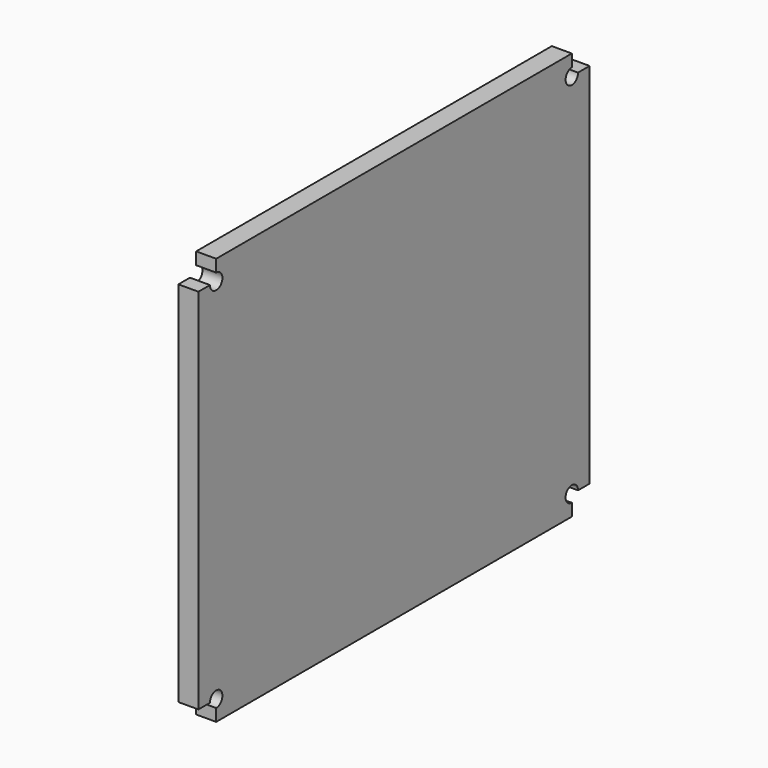
from build123d import *

# Parameters (mm, degrees)
F1_DEPTH = 9


# Not quite as in the source:
# - ends of sketch curves that miss each other by under 0.0002 mm in the source are joined


with BuildPart() as f1:
    # F0 (on Right) → F1 (new body)
    with BuildSketch(Plane.YZ):
        with BuildLine():
            Line((-71.5472308397, 116.6226820285), (-78.0472308397, 116.6226820285))
            Line((-78.0472308397, 116.6226820285), (-78.0472319707, -48.8313179715))
            Line((-78.0472319707, -48.8313179715), (-71.5472308397, -48.8313179715))
            ThreePointArc((-71.5472308397, -48.8313179715), (-65.5723571056, -46.3564442373), (-68.0472308397, -52.3313179715))
            Line((-68.0472308397, -52.3313179715), (-68.0472308397, -57.8313179715))
            Line((-68.0472308397, -57.8313179715), (31.9527691603, -57.8313179715))
            Line((31.9527691603, -57.8313179715), (131.9527668982, -57.8313179715))
            Line((131.9527668982, -57.8313179715), (131.9527668982, -52.3313179715))
            ThreePointArc((131.9527668982, -52.3313179715), (129.4778931641, -46.3564442373), (135.4527668982, -48.8313179715))
            Line((135.4527668982, -48.8313179715), (141.9527668982, -48.8313179715))
            Line((141.9527668982, -48.8313179715), (141.9527680293, 116.6226820285))
            Line((141.9527680293, 116.6226820285), (135.4527668982, 116.6226820285))
            ThreePointArc((135.4527668982, 116.6226820285), (129.4778931641, 114.1478082944), (131.9527668982, 120.1226820285))
            Line((131.9527668982, 120.1226820285), (131.9527668982, 125.6226820285))
            Line((131.9527668982, 125.6226820285), (31.9527668982, 125.6226820285))
            Line((31.9527668982, 125.6226820285), (-68.0472308397, 125.6226820285))
            Line((-68.0472308397, 125.6226820285), (-68.0472308397, 120.1226820285))
            ThreePointArc((-68.0472308397, 120.1226820285), (-65.5723571056, 114.1478082944), (-71.5472308397, 116.6226820285))
        make_face()
    extrude(amount=F1_DEPTH)


solid = f1.part
